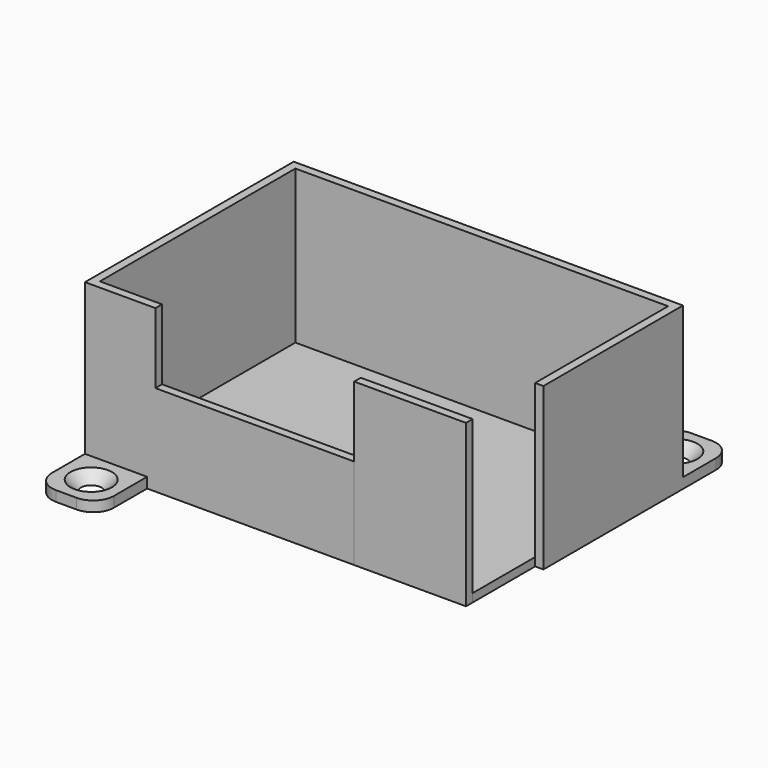
from build123d import *

# Parameters (mm, degrees)
F1_DEPTH = 39
F0_W     = 27
F0_H     = 2
F0_W_2   = 48
F2_DEPTH = 22
F3_DEPTH = 2
F0_R     = 2
F4_DEPTH = 2.5
F6_R     = 5


# Not quite as in the source:
# - a fillet or chamfer that OpenCascade refuses, or shapes differently, is made with other operations: its cross-section is extruded or revolved along the edge and cut away or added


with BuildPart() as f1:
    # F0 (on Top) → F1 (new body)
    with BuildSketch(Plane.XY):
        Polygon((10.8188620284, -66.1095576286), (10.8188620284, -7.1095576286), (100.8188620284, -7.1095576286), (100.8188620284, -47.2407341003), (102.8188620284, -47.2407341003), (102.8188620284, -7.5), (102.8188620284, -7.1095576286), (102.8188620284, -5.1095576286), (100.8188620284, -5.1095576286), (87.8188620284, -5.1095576286), (10.8188620284, -5.1095576286), (8.8188620284, -5.1095576286), (8.8188620284, -68.1095576286), (10.8188620284, -68.1095576286), (23.8188620284, -68.1095576286), (25.8188620284, -68.1095576286), (25.8188620284, -66.1095576286), align=None)
    extrude(amount=F1_DEPTH)

    # F0 (on Top) → F2 (join)
    with BuildSketch(Plane.XY):
        with Locations((49.8188620284, -67.1095576286)):
            Rectangle(F0_W_2, F0_H)
    extrude(amount=F2_DEPTH)

    # F0 (on Top) → F3 (join)
    with BuildSketch(Plane.XY):
        Polygon((100.8188620284, -7.1095576286), (10.8188620284, -7.1095576286), (10.8188620284, -66.1095576286), (25.8188620284, -66.1095576286), (73.8188620284, -66.1095576286), (100.8188620284, -66.1095576286), (100.8188620284, -47.2407341003), align=None)
    extrude(amount=F3_DEPTH)

    # F0 (on Top) → F4 (join)
    with BuildSketch(Plane.XY):
        Polygon((23.8188620284, -83.1095576286), (23.8188620284, -68.1095576286), (10.8188620284, -68.1095576286), (8.8188620284, -68.1095576286), (8.8188620284, -83.1095576286), align=None)
        with Locations((16.3188620284, -75.6095576286)):
            Circle(F0_R, mode=Mode.SUBTRACT)
        Polygon((100.8188620284, -5.1095576286), (102.8188620284, -5.1095576286), (102.8188620284, 9.8904423714), (87.8188620284, 9.8904423714), (87.8188620284, -5.1095576286), align=None)
        with Locations((95.3188620284, 2.3904423714)):
            Circle(F0_R, mode=Mode.SUBTRACT)
    extrude(amount=F4_DEPTH)

    # F5: chamfer of 3 on 2 edges, made by hand

    # F5_s1 → F5_t2 (revolve, cut)
    with BuildSketch(Plane.XZ.offset(75.6095576286)):
        Polygon((18.3188620284, -0.5), (21.3188620284, 2.5), (18.3188620284, 2.5), align=None)
    revolve(axis=Axis((16.3188620284, -75.6095576286, 2.5), (0, 0, 1)), mode=Mode.SUBTRACT)

    # F5_s3 → F5_t4 (revolve, cut)
    with BuildSketch(Plane.XZ.offset(-2.3904423714)):
        Polygon((100.3188620284, 2.5), (97.3188620284, -0.5), (97.3188620284, 2.5), align=None)
    revolve(axis=Axis((95.3188620284, 2.3904423714, 2.5), (0, 0, 1)), mode=Mode.SUBTRACT)

    # F6
    f6_edges = [f1.edges().sort_by_distance(p)[0] for p in [
        (102.818862, 9.890442, 1.25),
        (87.818862, 9.890442, 1.25),
        (8.818862, -83.109558, 1.25),
        (23.818862, -83.109558, 1.25),
    ]]
    fillet(f6_edges, radius=F6_R)


with BuildPart() as f1b:
    # F0 (on Top) → F1, piece 2 (new body)
    with BuildSketch(Plane.XY):
        with Locations((87.3188620284, -67.1095576286)):
            Rectangle(F0_W, F0_H)
    extrude(amount=F1_DEPTH)


solid = Compound([f1.part, f1b.part])
